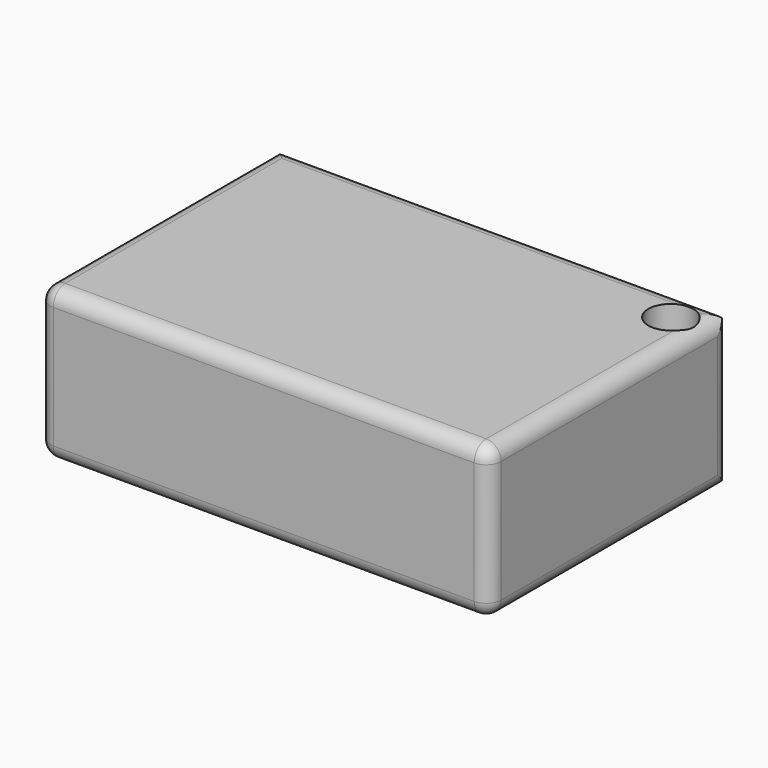
from build123d import *

# Parameters (mm, degrees)
F0_W         = 300
F0_H         = 200
F0_R         = 15
F1_DEPTH     = 101.12201
F2_T1_DEPTH  = 151.12201
F2_T3_DEPTH  = 350
F3_T1_DEPTH  = 205
F3_T3_DEPTH  = 280
F3_T5_DEPTH  = 81.12201
F3_S9_W      = 10.2
F3_S9_H      = 10.2
F3_T10_DEPTH = 10.2
F3_S15_W     = 10.2
F3_S15_H     = 10.2
F3_T16_DEPTH = 10.2
F3_S21_W     = 10.2
F3_S21_H     = 10.2
F3_T22_DEPTH = 10.2
F3_S27_W     = 10.2
F3_S27_H     = 10.2
F3_T28_DEPTH = 10.2


# Not quite as in the source:
# - a fillet or chamfer that OpenCascade refuses, or shapes differently, is made with other operations: its cross-section is extruded or revolved along the edge and cut away or added


with BuildPart() as f1:
    # F0 (on Top) → F1 (new body)
    with BuildSketch(Plane.XY):
        with Locations((0.0711865723, 30.1078906848)):
            Rectangle(F0_W, F0_H)
        with Locations((129.520341754, 106.8741083145)):
            Circle(F0_R, mode=Mode.SUBTRACT)
    extrude(amount=F1_DEPTH)

    # F2: fillet of radius 10 on 4 edges, made by hand

    # F2_s2 → F2_t1 (cut)
    with BuildSketch(Plane.XY.offset(-25)):
        with BuildLine():
            ThreePointArc((-139.9288134277, 130.1078906848), (-146.9998812396, 127.1789584967), (-149.9288134277, 120.1078906848))
            Line((-149.9288134277, 120.1078906848), (-149.9288134277, 130.1078906848))
            Line((-149.9288134277, 130.1078906848), (-139.9288134277, 130.1078906848))
        make_face()
        with BuildLine():
            ThreePointArc((140.0711865723, 130.1078906848), (147.1422543842, 127.1789584967), (150.0711865723, 120.1078906848))
            Line((150.0711865723, 120.1078906848), (150.0711865723, 130.1078906848))
            Line((150.0711865723, 130.1078906848), (140.0711865723, 130.1078906848))
        make_face()
    extrude(amount=F2_T1_DEPTH, mode=Mode.SUBTRACT)

    # F2_s4 → F2_t3 (cut)
    with BuildSketch(Plane.YZ.offset(-174.9288134277)):
        with BuildLine():
            ThreePointArc((130.1078906848, 10), (127.1789584967, 2.9289321881), (120.1078906848, 0))
            Line((120.1078906848, 0), (130.1078906848, 0))
            Line((130.1078906848, 0), (130.1078906848, 10))
        make_face()
        with BuildLine():
            ThreePointArc((130.1078906848, 91.12201), (127.1789584967, 98.1930778119), (120.1078906848, 101.12201))
            Line((120.1078906848, 101.12201), (130.1078906848, 101.12201))
            Line((130.1078906848, 101.12201), (130.1078906848, 91.12201))
        make_face()
    extrude(amount=F2_T3_DEPTH, mode=Mode.SUBTRACT)

    # F3: fillet of radius 10 on 13 edges, made by hand

    # F3_s2 → F3_t1 (cut)
    with BuildSketch(Plane.XZ.offset(-145.1078906848)):
        with BuildLine():
            ThreePointArc((-139.9288134277, 0), (-146.9998812396, 2.9289321881), (-149.9288134277, 10))
            Line((-149.9288134277, 10), (-149.9288134277, 0))
            Line((-149.9288134277, 0), (-139.9288134277, 0))
        make_face()
        with BuildLine():
            ThreePointArc((140.0711865723, 0), (147.1422543842, 2.9289321881), (150.0711865723, 10))
            Line((150.0711865723, 10), (150.0711865723, 0))
            Line((150.0711865723, 0), (140.0711865723, 0))
        make_face()
        with BuildLine():
            ThreePointArc((140.0711865723, 101.12201), (147.1422543842, 98.1930778119), (150.0711865723, 91.12201))
            Line((150.0711865723, 91.12201), (150.0711865723, 101.12201))
            Line((150.0711865723, 101.12201), (140.0711865723, 101.12201))
        make_face()
        with BuildLine():
            ThreePointArc((-149.9288134277, 91.12201), (-146.9998812396, 98.1930778119), (-139.9288134277, 101.12201))
            Line((-139.9288134277, 101.12201), (-149.9288134277, 101.12201))
            Line((-149.9288134277, 101.12201), (-149.9288134277, 91.12201))
        make_face()
    extrude(amount=F3_T1_DEPTH, mode=Mode.SUBTRACT)

    # F3_s4 → F3_t3 (cut)
    with BuildSketch(Plane.YZ.offset(-139.9288134277)):
        with BuildLine():
            ThreePointArc((-59.8921093152, 0), (-66.963177127, 2.9289321881), (-69.8921093152, 10))
            Line((-69.8921093152, 10), (-69.8921093152, 0))
            Line((-69.8921093152, 0), (-59.8921093152, 0))
        make_face()
        with BuildLine():
            ThreePointArc((-59.8921093152, 101.12201), (-66.963177127, 98.1930778119), (-69.8921093152, 91.12201))
            Line((-69.8921093152, 91.12201), (-69.8921093152, 101.12201))
            Line((-69.8921093152, 101.12201), (-59.8921093152, 101.12201))
        make_face()
    extrude(amount=F3_T3_DEPTH, mode=Mode.SUBTRACT)

    # F3_s6 → F3_t5 (cut)
    with BuildSketch(Plane.XY.offset(10)):
        with BuildLine():
            ThreePointArc((-149.9288134277, -59.8921093152), (-146.9998812396, -66.963177127), (-139.9288134277, -69.8921093152))
            Line((-139.9288134277, -69.8921093152), (-149.9288134277, -69.8921093152))
            Line((-149.9288134277, -69.8921093152), (-149.9288134277, -59.8921093152))
        make_face()
        with BuildLine():
            ThreePointArc((150.0711865723, -59.8921093152), (147.1422543842, -66.963177127), (140.0711865723, -69.8921093152))
            Line((140.0711865723, -69.8921093152), (150.0711865723, -69.8921093152))
            Line((150.0711865723, -69.8921093152), (150.0711865723, -59.8921093152))
        make_face()
    extrude(amount=F3_T5_DEPTH, mode=Mode.SUBTRACT)


with BuildPart() as f3_tool8:
    # F3_s9 → F3_t10 (new body)
    with BuildSketch(Plane.XZ.offset(59.8921093152)):
        with Locations((-145.0288134277, 4.9)):
            Rectangle(F3_S9_W, F3_S9_H)
    extrude(amount=F3_T10_DEPTH)

    # F3_s11 → F3_t12 (revolve, cut)
    with BuildSketch(Plane(origin=(-139.9288134277, -59.8921093152, 10), x_dir=(0.7071067812, 0, 0.7071067812), z_dir=(0.7071067812, 0, -0.7071067812))):
        with BuildLine():
            ThreePointArc((0, -10), (10, 0), (0, 10))
            Line((0, 10), (0, -10))
        make_face()
    revolve(axis=Axis((-139.9288134277, -59.8921093152, 10), (0, -1, 0)), mode=Mode.SUBTRACT)


with BuildPart() as f1_1:
    add(f1.part)

    # F3_t7: cut F3_tool8
    add(f3_tool8.part, mode=Mode.SUBTRACT)


with BuildPart() as f3_tool14:
    # F3_s15 → F3_t16 (new body)
    with BuildSketch(Plane.YZ.offset(140.0711865723)):
        with Locations((-64.9921093152, 4.9)):
            Rectangle(F3_S15_W, F3_S15_H)
    extrude(amount=F3_T16_DEPTH)

    # F3_s17 → F3_t18 (revolve, cut)
    with BuildSketch(Plane(origin=(140.0711865723, -59.8921093152, 10), x_dir=(0, 0.7071067812, 0.7071067812), z_dir=(0, 0.7071067812, -0.7071067812))):
        with BuildLine():
            ThreePointArc((0, -10), (10, 0), (0, 10))
            Line((0, 10), (0, -10))
        make_face()
    revolve(axis=Axis((140.0711865723, -59.8921093152, 10), (1, 0, 0)), mode=Mode.SUBTRACT)


with BuildPart() as f1_2:
    add(f1_1.part)

    # F3_t13: cut F3_tool14
    add(f3_tool14.part, mode=Mode.SUBTRACT)


with BuildPart() as f3_tool20:
    # F3_s21 → F3_t22 (new body)
    with BuildSketch(Plane.XY.offset(91.12201)):
        with Locations((-145.0288134277, -64.9921093152)):
            Rectangle(F3_S21_W, F3_S21_H)
    extrude(amount=F3_T22_DEPTH)

    # F3_s23 → F3_t24 (revolve, cut)
    with BuildSketch(Plane(origin=(-139.9288134277, -59.8921093152, 91.12201), x_dir=(0.7071067812, 0.7071067812, 0), z_dir=(0.7071067812, -0.7071067812, 0))):
        with BuildLine():
            ThreePointArc((0, -10), (10, 0), (0, 10))
            Line((0, 10), (0, -10))
        make_face()
    revolve(axis=Axis((-139.9288134277, -59.8921093152, 91.12201), (0, 0, 1)), mode=Mode.SUBTRACT)


with BuildPart() as f1_3:
    add(f1_2.part)

    # F3_t19: cut F3_tool20
    add(f3_tool20.part, mode=Mode.SUBTRACT)


with BuildPart() as f3_tool26:
    # F3_s27 → F3_t28 (new body)
    with BuildSketch(Plane.XY.offset(91.12201)):
        with Locations((145.1711865723, -64.9921093152)):
            Rectangle(F3_S27_W, F3_S27_H)
    extrude(amount=F3_T28_DEPTH)

    # F3_s29 → F3_t30 (revolve, cut)
    with BuildSketch(Plane(origin=(140.0711865723, -59.8921093152, 91.12201), x_dir=(-0.7071067812, 0.7071067812, 0), z_dir=(0.7071067812, 0.7071067812, 0))):
        with BuildLine():
            ThreePointArc((0, -10), (10, 0), (0, 10))
            Line((0, 10), (0, -10))
        make_face()
    revolve(axis=Axis((140.0711865723, -59.8921093152, 91.12201), (0, 0, 1)), mode=Mode.SUBTRACT)


with BuildPart() as f1_4:
    add(f1_3.part)

    # F3_t25: cut F3_tool26
    add(f3_tool26.part, mode=Mode.SUBTRACT)


solid = f1_4.part
